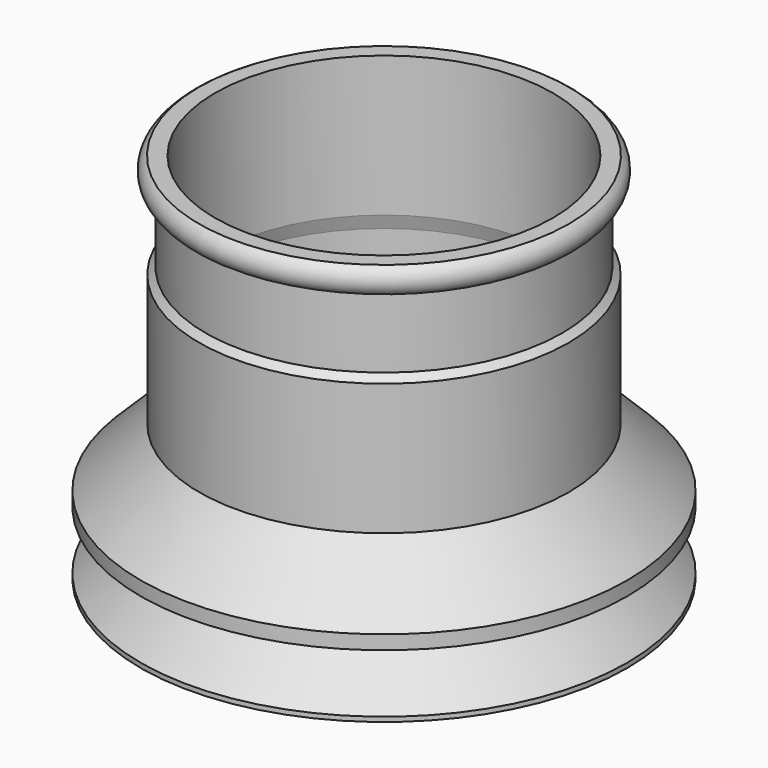
from build123d import *


# Not quite as in the source:
# - a feature names something its author has since deleted; it is built from what else it names


with BuildPart() as f1:
    # F0 (on Front) → F1 (revolve)
    with BuildSketch(Plane.XZ):
        with BuildLine():
            Line((52, -12.5), (39.5, 0))
            Line((39.5, 0), (52, 0))
            Line((52, 0), (52, 3))
            Line((52, 3), (39.5, 3))
            Line((39.5, 3), (39.5, 15.5))
            Line((39.5, 15.5), (39.5, 43.6252272915))
            Line((39.5, 43.6252272915), (38.1252272915, 45))
            Line((38.1252272915, 45), (38.1252272915, 60))
            ThreePointArc((38.1252272915, 60), (40.9990174252, 62.4871708245), (39.5482522386, 66))
            Line((39.5482522386, 66), (36.1252272915, 66))
            Line((36.1252272915, 66), (36.1252272915, 36))
            Line((36.1252272915, 36), (37, 33))
            Line((37, 33), (37, -1.0355339059))
            Line((37, -1.0355339059), (49.4644660941, -13.5))
            Line((49.4644660941, -13.5), (52, -13.5))
            Line((52, -13.5), (52, -12.5))
        make_face()
        Polygon((39.5, 3), (52, 3), (39.5, 15.5), align=None)
    revolve(axis=Axis((0, 0, 34.5994567809), (0, 0, -1)))


solid = f1.part
